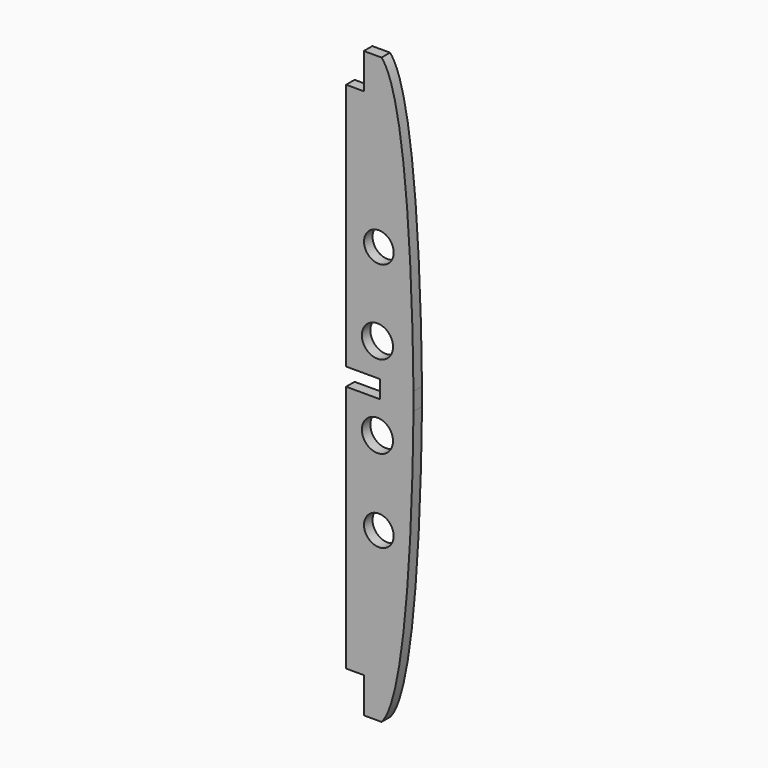
from build123d import *

# Parameters (mm, degrees)
F0_R     = 8.3591394984
F0_R_2   = 8.7902247906
F1_DEPTH = 6


# Not quite as in the source:
# - a feature names something its author has since deleted; it is built from what else it names


with BuildPart() as f1:
    # F0 (on Front) → F1 (new body)
    with BuildSketch(Plane.XZ):
        with BuildLine():
            Line((100.5853836174, -74.9584571321), (110.5853836174, -74.9584571321))
            add(Edge.make_bspline(
                [(110.5853836174, -74.9584571321), (126.6854561112, -57.248377389), (128.3848433658, 59.317552439), (128.5642162874, 85.0415428679)],
                knots=[0, 0, 0, 0, 148.4595862799, 148.4595862799, 148.4595862799, 148.4595862799], degree=3))
            Line((128.5642162874, 85.0415428679), (109.5853836174, 85.0415428679))
            Line((109.5853836174, 85.0415428679), (90.5853836174, 85.0415428679))
            Line((90.5853836174, 85.0415428679), (90.5853836174, -54.9584571321))
            Line((90.5853836174, -54.9584571321), (100.5853836174, -54.9584571321))
            Line((100.5853836174, -54.9584571321), (100.5853836174, -74.9584571321))
        make_face()
        with Locations((109.0683937073, 19.6757875151)):
            Circle(F0_R, mode=Mode.SUBTRACT)
        with Locations((108.2727760077, 66.6170529789)):
            Circle(F0_R_2, mode=Mode.SUBTRACT)
        with BuildLine():
            add(Edge.make_bspline(
                [(128.5642162874, 85.0415428679), (128.5853836174, 88.0771637948), (128.5853836174, 89.8477431573), (128.5853836174, 90.0415428679)],
                knots=[148.4595862799, 148.4595862799, 148.4595862799, 148.4595862799, 165.9789143235, 165.9789143235, 165.9789143235, 165.9789143235], degree=3))
            Line((128.5853836174, 90.0415428679), (109.5853836174, 90.0415428679))
            Line((109.5853836174, 90.0415428679), (109.5853836174, 85.0415428679))
            Line((109.5853836174, 85.0415428679), (128.5642162874, 85.0415428679))
        make_face()
        with BuildLine():
            Line((109.5853836174, 90.0415428679), (128.5853836174, 90.0415428679))
            add(Edge.make_bspline(
                [(128.5642162874, 95.0415428679), (128.5853836174, 92.005921941), (128.5853836174, 90.2353425785), (128.5853836174, 90.0415428679)],
                knots=[148.4595862799, 148.4595862799, 148.4595862799, 148.4595862799, 165.9789143235, 165.9789143235, 165.9789143235, 165.9789143235], degree=3))
            Line((128.5642162874, 95.0415428679), (109.5853836174, 95.0415428679))
            Line((109.5853836174, 95.0415428679), (109.5853836174, 90.0415428679))
        make_face()
        with BuildLine():
            Line((109.5853836174, 95.0415428679), (128.5642162874, 95.0415428679))
            add(Edge.make_bspline(
                [(110.5853836174, 255.0415428679), (126.6854561112, 237.3314631248), (128.3848433658, 120.7655332968), (128.5642162874, 95.0415428679)],
                knots=[0, 0, 0, 0, 148.4595862799, 148.4595862799, 148.4595862799, 148.4595862799], degree=3))
            Line((110.5853836174, 255.0415428679), (100.5853836174, 255.0415428679))
            Line((100.5853836174, 255.0415428679), (100.5853836174, 235.0415428679))
            Line((100.5853836174, 235.0415428679), (90.5853836174, 235.0415428679))
            Line((90.5853836174, 235.0415428679), (90.5853836174, 95.0415428679))
            Line((90.5853836174, 95.0415428679), (109.5853836174, 95.0415428679))
        make_face()
        with Locations((108.2727760077, 113.4660327569)):
            Circle(F0_R_2, mode=Mode.SUBTRACT)
        with Locations((109.0683937073, 160.4072982207)):
            Circle(F0_R, mode=Mode.SUBTRACT)
    extrude(amount=F1_DEPTH)


solid = f1.part
